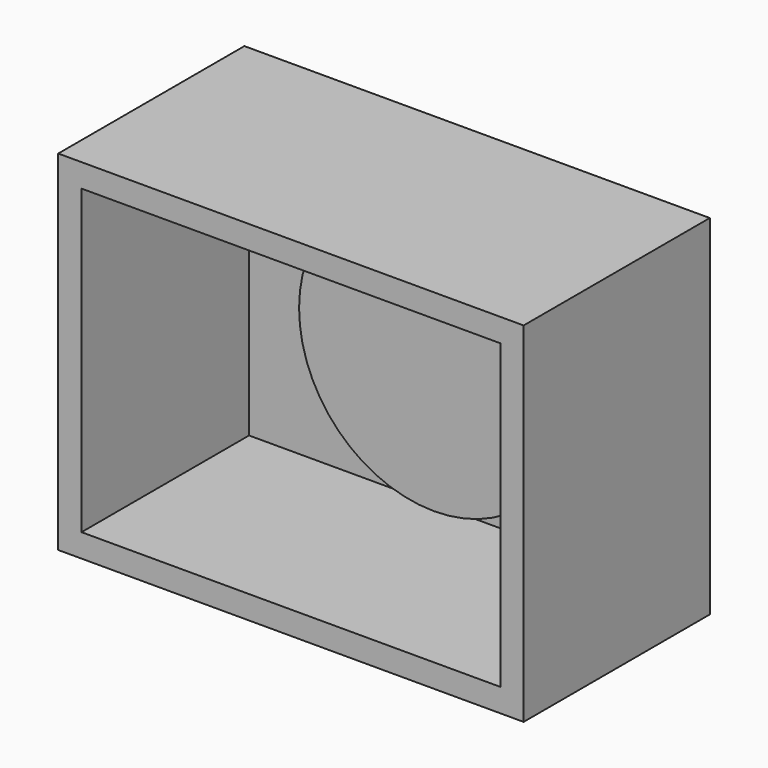
from build123d import *

# Parameters (mm, degrees)
F0_W     = 40
F0_H     = 30
F1_DEPTH = 20
F2_T     = -2
F3_R     = 11.6056457338
F4_DEPTH = 2


# Not quite as in the source:
# - the program builds the solid bodies; features that only make, move or delete a surface that nothing else refers to are left out


with BuildPart() as f1:
    # F0 (on Front) → F1 (new body)
    with BuildSketch(Plane.XZ):
        with Locations((-20, 15)):
            Rectangle(F0_W, F0_H)
    extrude(amount=F1_DEPTH)

    # F2
    f2_openings = [f1.faces().sort_by_distance(p)[0] for p in [
        (-20, -20, 15),
    ]]
    offset(amount=F2_T, openings=f2_openings)


with BuildPart() as f4:
    # F3 (on face) → F4 (new body)
    with BuildSketch(Plane.XZ.offset(2)):
        with Locations((-20.4928908497, 14.3788000569)):
            Circle(F3_R)
    extrude(amount=F4_DEPTH)


solid = Compound([f1.part, f4.part])
